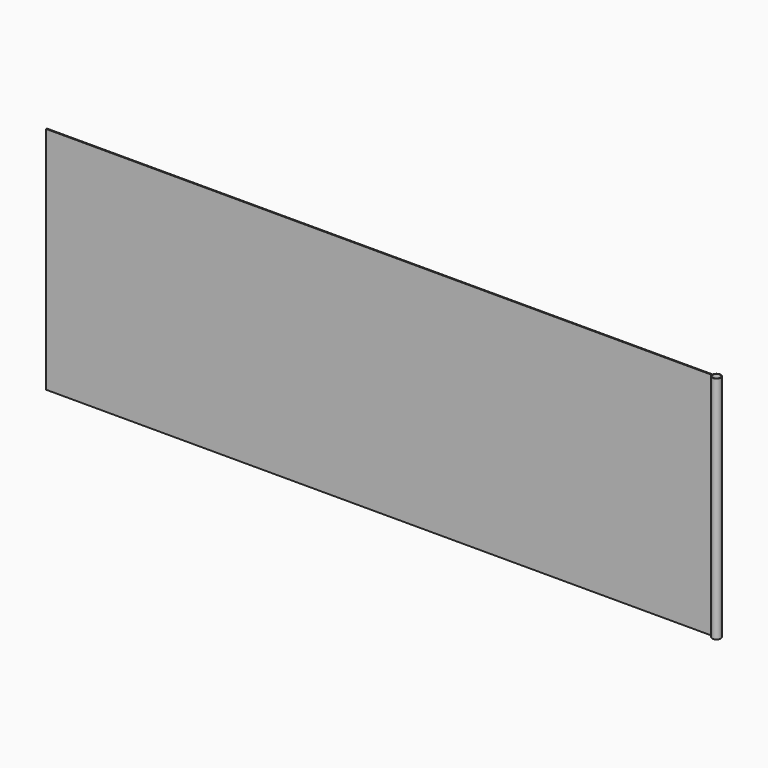
from build123d import *

# Parameters (mm, degrees)
F1_DEPTH = 1524
F2_T     = -2.54


with BuildPart() as f1:
    # F0 (on Top) → F1 (new body)
    with BuildSketch(Plane.XY):
        with BuildLine():
            ThreePointArc((2265.68, 0), (2237.74, 27.94), (2209.8, 0))
            ThreePointArc((2209.8, 0), (2237.74, -27.94), (2265.68, 0))
        make_face()
    extrude(amount=F1_DEPTH)

    # F2
    f2_openings = [f1.faces().sort_by_distance(p)[0] for p in [
        (2237.74, 0, 1524),
    ]]
    offset(amount=F2_T, openings=f2_openings)


with BuildPart() as f1b:
    # F0 (on Top) → F1, piece 2 (new body)
    with BuildSketch(Plane.XY):
        Polygon((2209.8, 0), (2209.8, 3.175), (-2209.8, 3.175), (-2209.8, -3.175), (2209.8, -3.175), align=None)
    extrude(amount=F1_DEPTH)


solid = Compound([f1.part, f1b.part])
